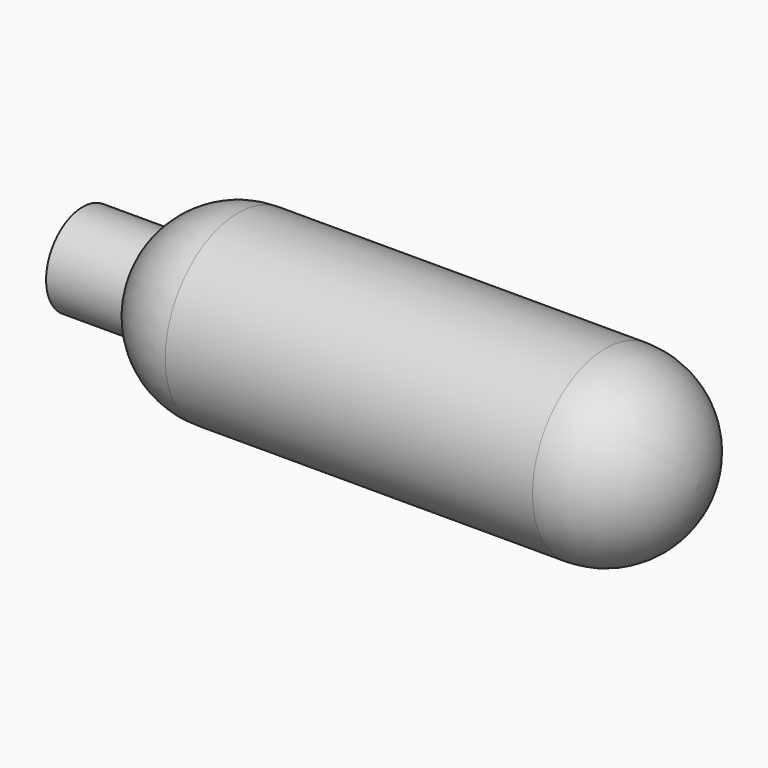
from build123d import *

# Parameters (mm, degrees)
F3_R = 9.4996


# Not quite as in the source:
# - a fillet or chamfer that OpenCascade refuses, or shapes differently, is made with other operations: its cross-section is extruded or revolved along the edge and cut away or added


with BuildPart() as f1:
    # F0 (on Front) → F1 (revolve)
    with BuildSketch(Plane.XZ):
        Polygon((0, 4.7723002699), (0, 0), (64, 0), (64, 9.5), (8, 9.5), (8, 4.7723002699), align=None)
    revolve(axis=Axis((32, 0, 0), (-1, 0, 0)))

    # F2: fillet of radius 9.4996 on 1 edges, made by hand

    # F2_s1 → F2_t2 (revolve, cut)
    with BuildSketch(Plane.XZ):
        with BuildLine():
            ThreePointArc((16.2140956882, 9.5), (11.4753587068, 8.2336722524), (8, 4.7723002699))
            Line((8, 4.7723002699), (8, 9.5))
            Line((8, 9.5), (16.2140956882, 9.5))
        make_face()
    revolve(axis=Axis((8, 0, 0), (-1, 0, 0)), mode=Mode.SUBTRACT)

    # F3
    f3_edges = [f1.edges().sort_by_distance(p)[0] for p in [
        (64, 0, -9.5),
    ]]
    fillet(f3_edges, radius=F3_R)


solid = f1.part
